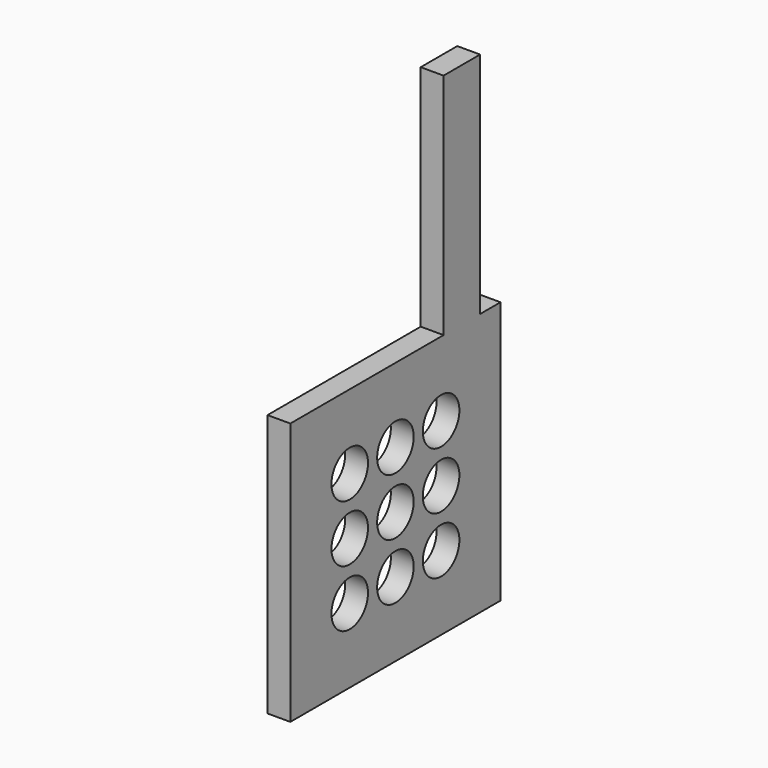
from build123d import *

# Parameters (mm, degrees)
F0_R     = 1
F1_DEPTH = 1


# Not quite as in the source:
# - a feature names something its author has since deleted; it is built from what else it names


with BuildPart() as f1:
    # F0 (on Right) → F1 (new body)
    with BuildSketch(Plane.YZ):
        Polygon((8.384144865, 0), (0, 0), (0, -11.5), (11.5, -11.5), (11.5, 0), (10.384144865, 0), (10.384144865, 10), (8.384144865, 10), align=None)
        with Locations((3.25, -8.25)):
            Circle(F0_R, mode=Mode.SUBTRACT)
        with Locations((3.25, -5.75)):
            Circle(F0_R, mode=Mode.SUBTRACT)
        with Locations((3.25, -3.25)):
            Circle(F0_R, mode=Mode.SUBTRACT)
        with Locations((5.75, -8.25)):
            Circle(F0_R, mode=Mode.SUBTRACT)
        with Locations((8.25, -8.25)):
            Circle(F0_R, mode=Mode.SUBTRACT)
        with Locations((5.75, -5.75)):
            Circle(F0_R, mode=Mode.SUBTRACT)
        with Locations((8.25, -5.75)):
            Circle(F0_R, mode=Mode.SUBTRACT)
        with Locations((5.75, -3.25)):
            Circle(F0_R, mode=Mode.SUBTRACT)
        with Locations((8.25, -3.25)):
            Circle(F0_R, mode=Mode.SUBTRACT)
    extrude(amount=F1_DEPTH)


solid = f1.part
